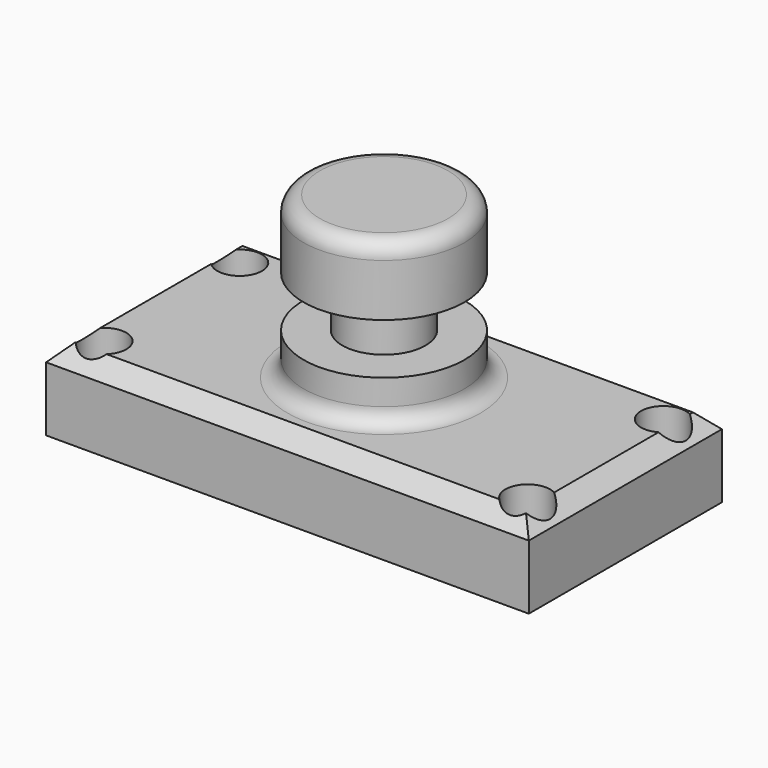
from build123d import *

# Parameters (mm, degrees)
F0_W         = 152.4
F0_H         = 76.2
F1_DEPTH     = 25.4
F2_R         = 7.0539826123
F3_DEPTH     = 25.401
F4_W         = 25.4
F4_H         = 50.8
F6_W         = 18.2314971462
F6_H         = 16.024235636
F9_R         = 5.08
F10_T1_DEPTH = 178.5282991577
F10_T3_DEPTH = 102.3282991577


# Not quite as in the source:
# - a fillet or chamfer that OpenCascade refuses, or shapes differently, is made with other operations: its cross-section is extruded or revolved along the edge and cut away or added


with BuildPart() as f1:
    # F0 (on Top) → F1 (new body)
    with BuildSketch(Plane.XY):
        Rectangle(F0_W, F0_H)
    extrude(amount=F1_DEPTH)

    # F2 (on face) → F3 (cut, through all)
    with BuildSketch(Plane.XY.offset(25.4)):
        with Locations((67.723274231, 25.5973488092)):
            Circle(F2_R)
        with Locations((-66.04, 25.5973488092)):
            Circle(F2_R)
        with Locations((-66.04, -27.94)):
            Circle(F2_R)
        with Locations((67.723274231, -27.94)):
            Circle(F2_R)
    extrude(amount=-F3_DEPTH, mode=Mode.SUBTRACT)

    # F4 (on Front) → F5 (revolve)
    with BuildSketch(Plane.XZ):
        with Locations((12.7, 50.8)):
            Rectangle(F4_W, F4_H)
    revolve(axis=Axis((0, 0, 50.8), (0, 0, 1)))

    # F6 (on Front) → F8 (revolve, cut)
    with BuildSketch(Plane.XZ):
        with Locations((22.2315485589, 46.5468037874)):
            Rectangle(F6_W, F6_H)
    revolve(axis=Axis((0, 0, 32.2526581585), (0, 0, 1)), mode=Mode.SUBTRACT)

    # F9
    f9_edges = [f1.edges().sort_by_distance(p)[0] for p in [
        (-25.4, 0, 76.2),
        (-25.4, 0, 25.4),
    ]]
    fillet(f9_edges, radius=F9_R)

    # F10: chamfer of 5.08 on 4 edges, made by hand

    # F10_s2 → F10_t1 (cut)
    with BuildSketch(Plane.YZ.offset(-89.2641495789)):
        Polygon((-33.02, 25.4), (-38.1, 20.32), (-38.1, 25.4), align=None)
        Polygon((33.02, 25.4), (38.1, 20.32), (38.1, 25.4), align=None)
    extrude(amount=F10_T1_DEPTH, mode=Mode.SUBTRACT)

    # F10_s4 → F10_t3 (cut)
    with BuildSketch(Plane.XZ.offset(-51.1641495789)):
        Polygon((71.12, 25.4), (76.2, 20.32), (76.2, 25.4), align=None)
        Polygon((-71.12, 25.4), (-76.2, 20.32), (-76.2, 25.4), align=None)
    extrude(amount=F10_T3_DEPTH, mode=Mode.SUBTRACT)


solid = f1.part
